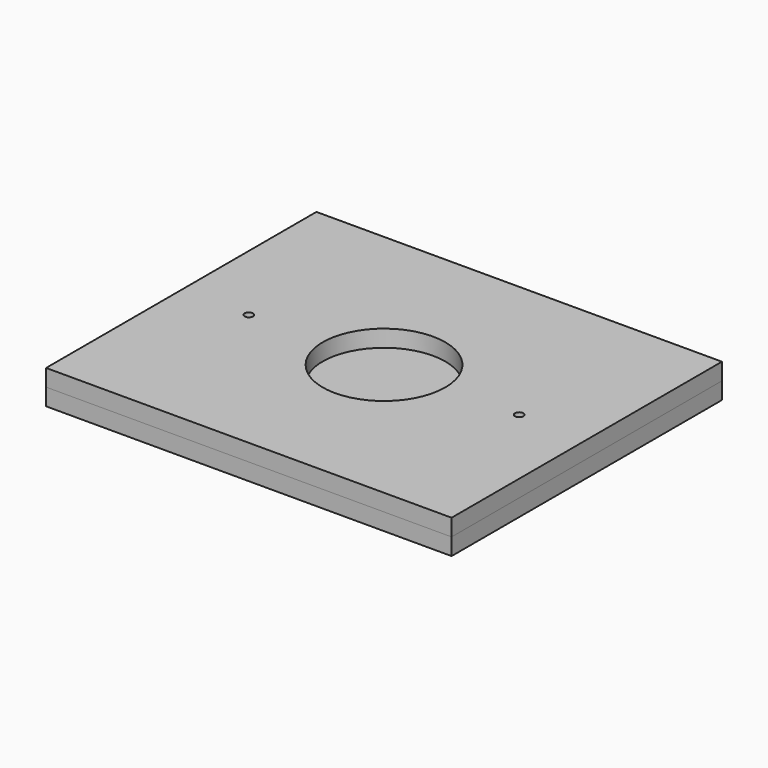
from build123d import *

# Parameters (mm, degrees)
F0_W     = 304.8
F0_H     = 254
F1_DEPTH = 6.35
F2_DEPTH = 12.7
F3_R     = 46.0375
F4_DEPTH = 25.401
F5_R     = 12.7
F6_DEPTH = 25.4
F7_R     = 3.175
F8_DEPTH = 25.401


with BuildPart() as f1:
    # F0 (on Top) → F1 (new body, symmetric)
    with BuildSketch(Plane.XY):
        Rectangle(F0_W, F0_H)
    extrude(amount=F1_DEPTH, both=True)


with BuildPart() as f2:
    # F2 (new): a face of the model
    f2_faces = [f1.part.faces().sort_by_distance(p)[0] for p in [
        (0, 0, 6.35),
    ]]
    extrude(f2_faces, amount=F2_DEPTH)

    # F3 (on face) → F4 (cut, through all)
    with BuildSketch(Plane.XY.offset(19.05)):
        Circle(F3_R)
    extrude(amount=-F4_DEPTH, mode=Mode.SUBTRACT)

    # F7 (on face) → F8 (cut, through all)
    with BuildSketch(Plane.XY.offset(19.05)):
        with Locations((-101.6, 0)):
            Circle(F7_R)
        with Locations((101.6, 0)):
            Circle(F7_R)
    extrude(amount=-F8_DEPTH, mode=Mode.SUBTRACT)


with BuildPart() as f1_1:
    add(f1.part)

    # F5 (on face) → F6 (cut)
    with BuildSketch(Plane(origin=(0, 0, -6.35), x_dir=(1, 0, 0), z_dir=(0, 0, -1))):
        with Locations((-101.6, 0)):
            Circle(F5_R)
        with Locations((101.6, 0)):
            Circle(F5_R)
    extrude(amount=-F6_DEPTH, mode=Mode.SUBTRACT)


solid = Compound([f2.part, f1_1.part])
